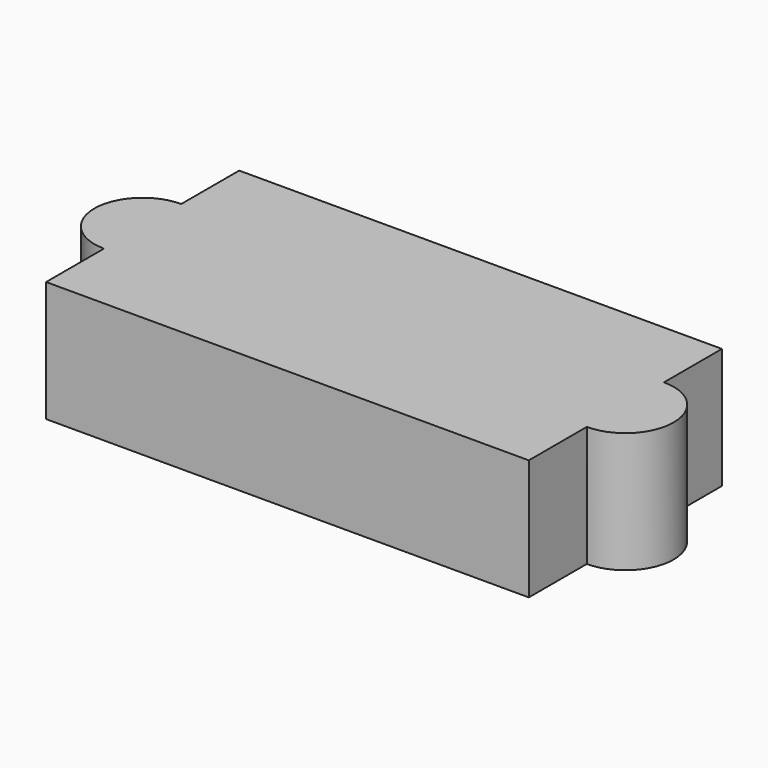
from build123d import *

# Parameters (mm, degrees)
F0_W     = 100
F0_H     = 50
F1_DEPTH = 25
F2_R     = 10
F3_DEPTH = 25


# Not quite as in the source:
# - a pattern or mirror of a feature is missing from the dataset's text; its kind, count and spacing are read off the source's solid


with BuildPart() as f1:
    # F0 (on Top) → F1 (new body)
    with BuildSketch(Plane.XY):
        with Locations((0, 25)):
            Rectangle(F0_W, F0_H)
    extrude(amount=F1_DEPTH)

    # F2 (on face) → F3 (join, through all)
    with BuildSketch(Plane.XY.offset(25)):
        with Locations((-50, 25)):
            Circle(F2_R)
    f3 = extrude(amount=-F3_DEPTH)

    # F3_copies: F3 across plane
    add(f3.mirror(Plane(origin=(0, 0, 0), x_dir=(0, 0, 1), z_dir=(1, 0, 0))))


solid = f1.part
